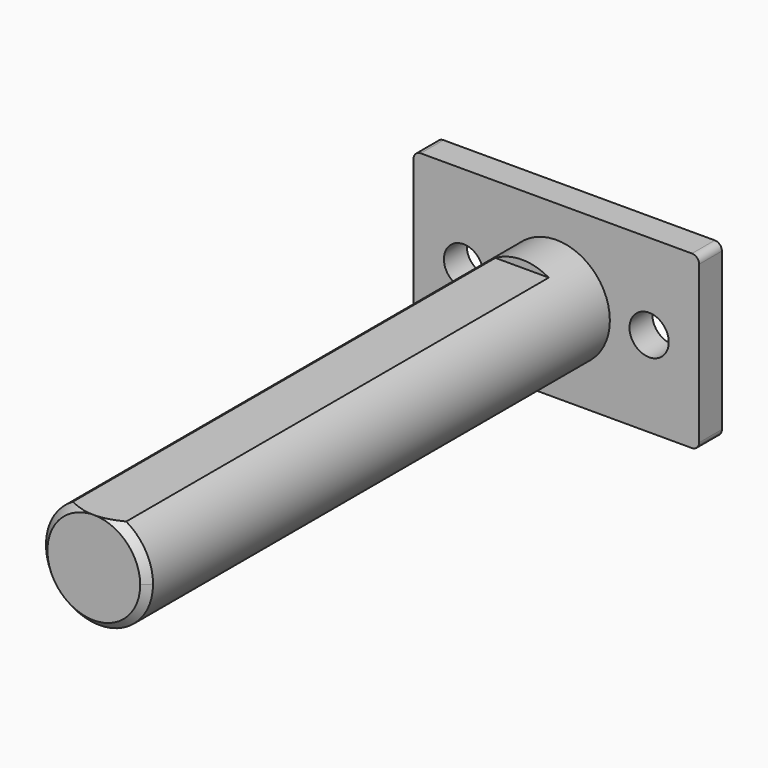
from build123d import *

# Parameters (mm, degrees)
F0_W      = 40
F0_H      = 24
F0_R      = 7.5
F1_DEPTH  = 4
F2_DEPTH  = 85
F4_D      = 5.5
F6_DEPTH  = 75
F7_R      = 1
F8_SIZE2  = 0.99999
F8_SIZE   = 0.99999
F9_R      = 7.5
F10_DEPTH = 2


# Not quite as in the source:
# - a fillet or chamfer is up to 0.001 mm smaller than in the source, because OpenCascade refuses the exact size


with BuildPart() as f1:
    # F0 (on Front) → F1 (new body)
    with BuildSketch(Plane.XZ):
        Rectangle(F0_W, F0_H)
        Circle(F0_R, mode=Mode.SUBTRACT)
    extrude(amount=F1_DEPTH)

    # F0 (on Front) → F2 (join)
    with BuildSketch(Plane.XZ):
        Circle(F0_R)
    extrude(amount=F2_DEPTH)

    # F4 (through all)
    with Locations(Plane.XZ.offset(4)):
        with Locations((-13, 0), (13, 0)):
            Hole(F4_D / 2)

    # F5 (on face) → F6 (cut)
    with BuildSketch(Plane.XZ.offset(85)):
        with BuildLine():
            Line((8.4905531257, 12.6322833821), (-12.126554407, 6.5))
            Line((-12.126554407, 6.5), (-3.7416573868, 6.5))
            ThreePointArc((-3.7416573868, 6.5), (0, 7.5), (3.7416573868, 6.5))
            Line((3.7416573868, 6.5), (18.1320688201, 6.5))
            Line((18.1320688201, 6.5), (8.4905531257, 12.6322833821))
        make_face()
        with BuildLine():
            ThreePointArc((3.7416573868, 6.5), (0, 7.5), (-3.7416573868, 6.5))
            Line((-3.7416573868, 6.5), (3.7416573868, 6.5))
        make_face()
    extrude(amount=-F6_DEPTH, mode=Mode.SUBTRACT)

    # F7
    f7_edges = [f1.edges().sort_by_distance(p)[0] for p in [
        (-20, -2, 12),
        (20, -2, 12),
        (20, -2, -12),
        (-20, -2, -12),
    ]]
    fillet(f7_edges, radius=F7_R)

    # F8 (size 1 and 1 in the source; OpenCascade refuses exactly that, so slightly less here)
    f8_edges = [f1.edges().sort_by_distance(p)[0] for p in [
        (-3.754169, -85, -6.492782),
        (6.492782, -85, 3.754169),
    ]]
    chamfer(f8_edges, length=F8_SIZE, length2=F8_SIZE2)

    # F9 (on face) → F10 (cut)
    with BuildSketch(Plane(origin=(0, 0, 0), x_dir=(-1, 0, 0), z_dir=(0, 1, 0))):
        Circle(F9_R)
    extrude(amount=-F10_DEPTH, mode=Mode.SUBTRACT)


solid = f1.part
